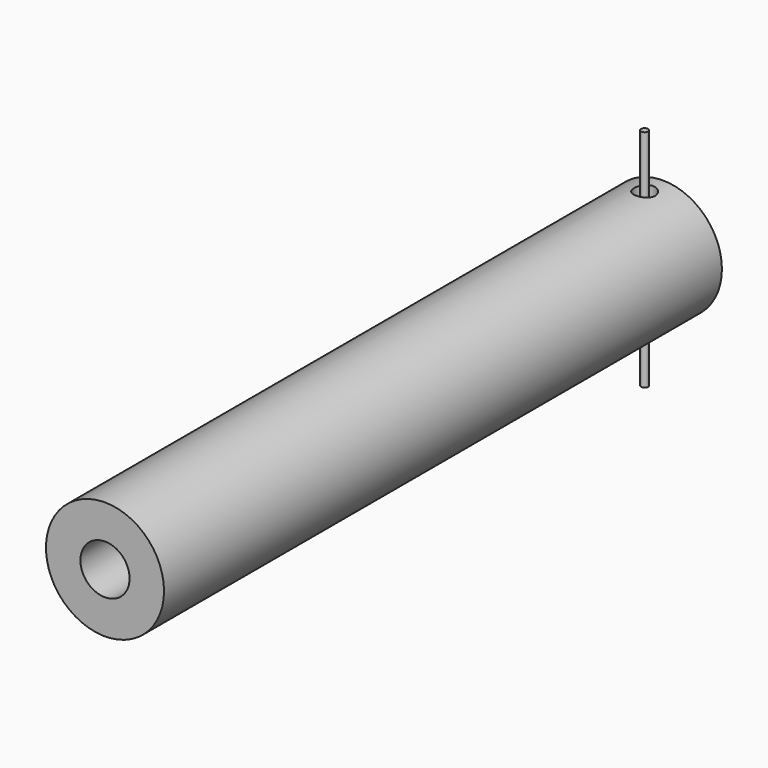
from build123d import *

# Parameters (mm, degrees)
F0_R      = 53.34
F0_R_2    = 22.225
F1_DEPTH  = 20.6375
F6_DEPTH  = 609.6
F5_R      = 9.525
F5_R_2    = 3.302
F7_DEPTH  = 19.05
F8_DEPTH  = 32.3616602869
F4_R      = 9.525
F4_R_2    = 3.302
F9_DEPTH  = 19.05
F10_DEPTH = 32.3616602869
F13_W     = 2.032
F13_H     = 3.556
F15_R     = 3.175
F16_DEPTH = 101.6


# Not quite as in the source:
# - the program builds the solid bodies; features that only make, move or delete a surface that nothing else refers to are left out


with BuildPart() as f1:
    # F0 (on Front) → F1 (new body)
    with BuildSketch(Plane.XZ):
        Circle(F0_R)
        Circle(F0_R_2, mode=Mode.SUBTRACT)
    extrude(amount=-F1_DEPTH)

    # F0 (on Front) → F6 (join)
    with BuildSketch(Plane.XZ):
        Circle(F0_R)
        Circle(F0_R_2, mode=Mode.SUBTRACT)
    extrude(amount=F6_DEPTH)

    # F5 (on offset) → F7 (cut)
    with BuildSketch(Plane.XY.offset(-53.34)):
        Circle(F5_R)
        Circle(F5_R_2, mode=Mode.SUBTRACT)
        Circle(F5_R_2)
    extrude(amount=F7_DEPTH, mode=Mode.SUBTRACT)

    # F5 (on offset) → F8 (cut, up to face)
    with BuildSketch(Plane.XY.offset(-53.34)):
        Circle(F5_R_2)
    extrude(amount=F8_DEPTH, mode=Mode.SUBTRACT)

    # F4 (on offset) → F9 (cut)
    with BuildSketch(Plane.XY.offset(53.34)):
        Circle(F4_R)
        Circle(F4_R_2, mode=Mode.SUBTRACT)
        Circle(F4_R_2)
    extrude(amount=-F9_DEPTH, mode=Mode.SUBTRACT)

    # F4 (on offset) → F10 (cut, up to face)
    with BuildSketch(Plane.XY.offset(53.34)):
        Circle(F4_R_2)
    extrude(amount=-F10_DEPTH, mode=Mode.SUBTRACT)

    # F11 (on Right) → F12 (revolve, cut)
    with BuildSketch(Plane.YZ):
        Polygon((6.35, 34.29), (3.302, 34.29), (3.302, 29.21), align=None)
        Polygon((3.302, -29.21), (3.302, -34.29), (6.35, -34.29), align=None)
    revolve(axis=Axis((0, 0, 6.9711627439), (0, 0, 1)), mode=Mode.SUBTRACT)

    # F13 (on Top) → F14 (revolve, cut)
    with BuildSketch(Plane.XY):
        Polygon((-25.4254, 11.1125), (-22.225, 11.1125), (-22.225, 20.6375), (-25.4254, 20.6375), (-25.4254, 17.653), (-25.4254, 14.097), align=None)
        with Locations((-26.4414, 15.875)):
            Rectangle(F13_W, F13_H)
    revolve(axis=Axis((0, 5.55625, 0), (0, 1, 0)), mode=Mode.SUBTRACT)


with BuildPart() as f16:
    # F15 (on Top) → F16 (new body, symmetric)
    with BuildSketch(Plane.XY):
        Circle(F15_R)
    extrude(amount=F16_DEPTH, both=True)


solid = Compound([f1.part, f16.part])
